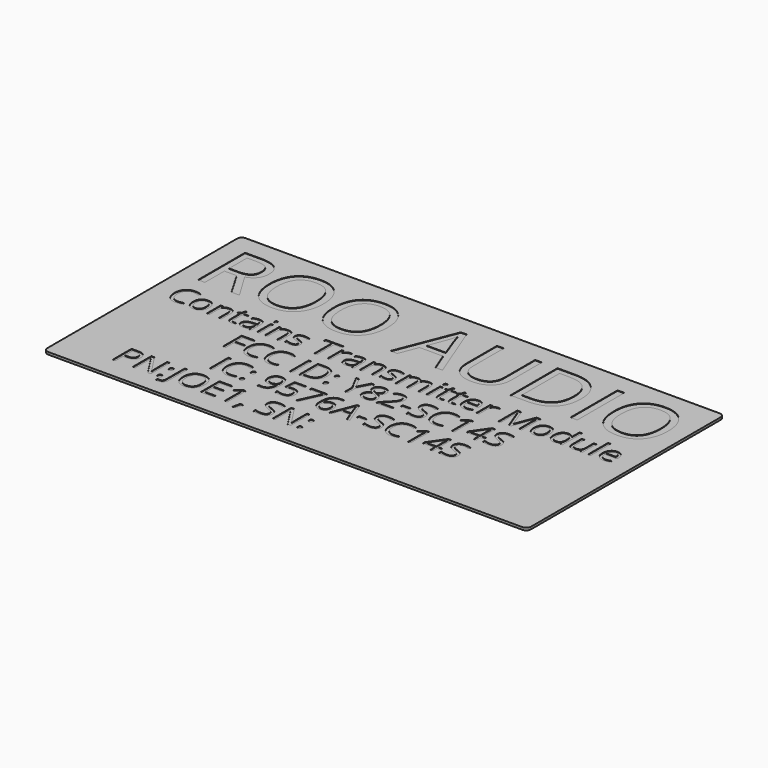
from build123d import *

# Parameters (mm, degrees)
F1_DEPTH       = 0.127
F3_TEXT_SIZE   = 1.7638888889
F3_TEXT_SIZE_2 = 4.4097222222
F4_DEPTH       = 0.0254


# Not quite as in the source:
# - Text() gives the source's letters only with a copy of the font that has no kerning and outlines rounded to 1/6400 em; it was checked with that copy


with BuildPart() as f1:
    # F0 (on Top) → F1 (new body)
    with BuildSketch(Plane.XY):
        with BuildLine():
            ThreePointArc((12.954, 6.35), (12.8796051224, 6.5296051224), (12.7, 6.604))
            Line((12.7, 6.604), (-12.7, 6.604))
            ThreePointArc((-12.7, 6.604), (-12.8796051224, 6.5296051224), (-12.954, 6.35))
            Line((-12.954, 6.35), (-12.954, -6.35))
            ThreePointArc((-12.954, -6.35), (-12.8796051224, -6.5296051224), (-12.7, -6.604))
            Line((-12.7, -6.604), (12.7, -6.604))
            ThreePointArc((12.7, -6.604), (12.8796051224, -6.5296051224), (12.954, -6.35))
            Line((12.954, -6.35), (12.954, 6.35))
        make_face()
    extrude(amount=F1_DEPTH)

    # F3 (on face) → F4 (cut)
    with BuildSketch(Plane.XY.offset(0.127)):
        with Locations((-12.0368880208, 0.254)):
            Text('Contains Transmitter Module', F3_TEXT_SIZE, font='Open Sans', text_align=(TextAlign.LEFT, TextAlign.BOTTOM))
        with Locations((-7.4839876302, -1.651)):
            Text('FCC ID: Y82-SC14S', F3_TEXT_SIZE, font='Open Sans', text_align=(TextAlign.LEFT, TextAlign.BOTTOM))
        with Locations((-6.672874349, -3.556)):
            Text('IC: 9576A-SC14S', F3_TEXT_SIZE, font='Open Sans', text_align=(TextAlign.LEFT, TextAlign.BOTTOM))
        with Locations((-12.324899435, 2.413)):
            Text('ROO AUDIO', F3_TEXT_SIZE_2, font='Open Sans', text_align=(TextAlign.LEFT, TextAlign.BOTTOM))
        with Locations((-10.3366644965, -5.461)):
            Text('PN:JOE1, SN:', F3_TEXT_SIZE, font='Open Sans', text_align=(TextAlign.LEFT, TextAlign.BOTTOM))
    extrude(amount=-F4_DEPTH, mode=Mode.SUBTRACT)


solid = f1.part
